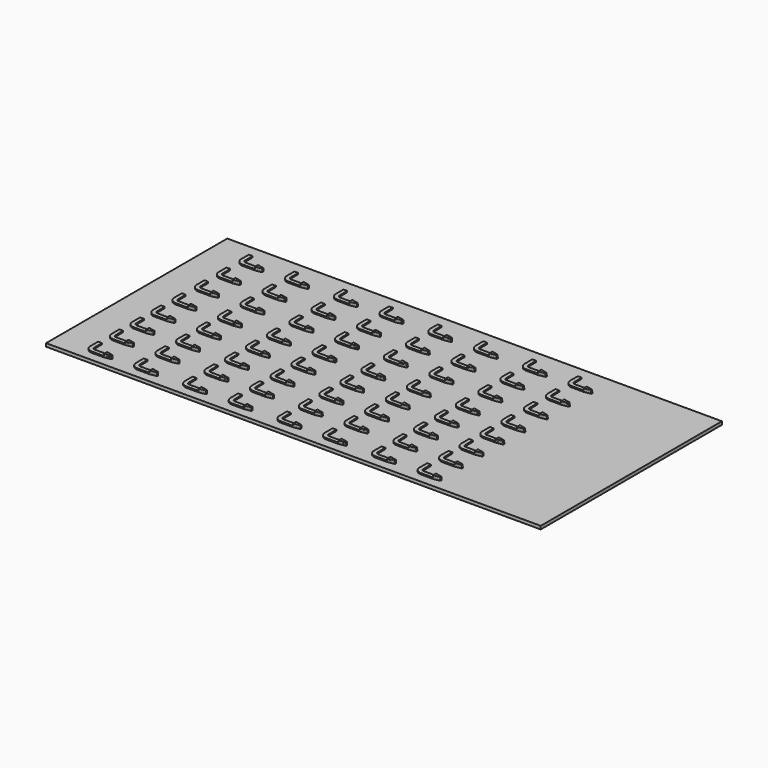
from build123d import *

# Parameters (mm, degrees)
F0_W     = 3907.0630930364
F0_H     = 1789.1258522868
F1_DEPTH = 25.4
F3_DEPTH = 10.16
F5_DEPTH = 7.62
F7_DEPTH = 7.62


# Not quite as in the source:
# - a feature names something its author has since deleted; it is built from what else it names


with BuildPart() as f1:
    # F0 (on Top) → F1 (new body)
    with BuildSketch(Plane.XY):
        with Locations((1503.1844954938, 391.7114809155)):
            Rectangle(F0_W, F0_H)
    extrude(amount=-F1_DEPTH)


with BuildPart() as f3:
    # F2 (on face) → F3 (new body)
    with BuildSketch(Plane.XY):
        with BuildLine():
            Line((0, 4.8675285652), (-51.4132715762, 16.0222817212))
            Line((-51.4132715762, 16.0222817212), (-149.2118090391, 16.0222817212))
            ThreePointArc((-149.2118090391, 16.0222817212), (-163.1179000848, 21.7124932059), (-169.0462678671, 35.5187356472))
            Line((-169.0462678671, 35.5187356472), (-170.3702134564, 112.54149833))
            Line((-170.3702134564, 112.54149833), (-199.8733133078, 112.0343690405))
            Line((-199.8733133078, 112.0343690405), (-199.8733133078, 35.5187356472))
            ThreePointArc((-199.8733133078, 35.5187356472), (-184.8444308949, 0.045176502), (-149.2118090391, -14.602586627))
            Line((-149.2118090391, -14.602586627), (-51.4132715762, -14.602586627))
            Line((-51.4132715762, -14.602586627), (0, -4.8675285652))
            Line((0, -4.8675285652), (0, 4.8675285652))
        make_face()
        with BuildLine():
            Line((0, 210.3862510994), (-51.4132715762, 221.5410042554))
            Line((-51.4132715762, 221.5410042554), (-149.2118090391, 221.5410042554))
            ThreePointArc((-149.2118090391, 221.5410042554), (-163.1179000848, 227.23121574), (-169.0462678671, 241.0374581814))
            Line((-169.0462678671, 241.0374581814), (-170.3702134564, 318.0602208642))
            Line((-170.3702134564, 318.0602208642), (-199.8733133078, 317.5530915746))
            Line((-199.8733133078, 317.5530915746), (-199.8733133078, 241.0374581814))
            ThreePointArc((-199.8733133078, 241.0374581814), (-184.8444308949, 205.5638990362), (-149.2118090391, 190.9161359072))
            Line((-149.2118090391, 190.9161359072), (-51.4132715762, 190.9161359072))
            Line((-51.4132715762, 190.9161359072), (0, 200.651193969))
            Line((0, 200.651193969), (0, 210.3862510994))
        make_face()
        with BuildLine():
            Line((0, -198.6540211365), (-51.4132715762, -187.4992679805))
            Line((-51.4132715762, -187.4992679805), (-149.2118090391, -187.4992679805))
            ThreePointArc((-149.2118090391, -187.4992679805), (-163.1179000848, -181.8090564958), (-169.0462678671, -168.0028140545))
            Line((-169.0462678671, -168.0028140545), (-170.3702134564, -90.9800513717))
            Line((-170.3702134564, -90.9800513717), (-199.8733133078, -91.4871806612))
            Line((-199.8733133078, -91.4871806612), (-199.8733133078, -168.0028140545))
            ThreePointArc((-199.8733133078, -168.0028140545), (-184.8444308949, -203.4763731996), (-149.2118090391, -218.1241363287))
            Line((-149.2118090391, -218.1241363287), (-51.4132715762, -218.1241363287))
            Line((-51.4132715762, -218.1241363287), (0, -208.3890782669))
            Line((0, -208.3890782669), (0, -198.6540211365))
        make_face()
        with BuildLine():
            Line((0, -409.4740850851), (-51.4132715762, -398.3193319291))
            Line((-51.4132715762, -398.3193319291), (-149.2118090391, -398.3193319291))
            ThreePointArc((-149.2118090391, -398.3193319291), (-163.1179000848, -392.6291204445), (-169.0462678671, -378.8228780031))
            Line((-169.0462678671, -378.8228780031), (-170.3702134564, -301.8001153203))
            Line((-170.3702134564, -301.8001153203), (-199.8733133078, -302.3072446099))
            Line((-199.8733133078, -302.3072446099), (-199.8733133078, -378.8228780031))
            ThreePointArc((-199.8733133078, -378.8228780031), (-184.8444308949, -414.2964371483), (-149.2118090391, -428.9442002773))
            Line((-149.2118090391, -428.9442002773), (-51.4132715762, -428.9442002773))
            Line((-51.4132715762, -428.9442002773), (0, -419.2091422155))
            Line((0, -419.2091422155), (0, -409.4740850851))
        make_face()
        with BuildLine():
            Line((0, 418.081481941), (-51.4132715762, 429.2362350971))
            Line((-51.4132715762, 429.2362350971), (-149.2118090391, 429.2362350971))
            ThreePointArc((-149.2118090391, 429.2362350971), (-163.1179000848, 434.9264465817), (-169.0462678671, 448.732689023))
            Line((-169.0462678671, 448.732689023), (-170.3702134564, 525.7554517058))
            Line((-170.3702134564, 525.7554517058), (-199.8733133078, 525.2483224163))
            Line((-199.8733133078, 525.2483224163), (-199.8733133078, 448.732689023))
            ThreePointArc((-199.8733133078, 448.732689023), (-184.8444308949, 413.2591298779), (-149.2118090391, 398.6113667488))
            Line((-149.2118090391, 398.6113667488), (-51.4132715762, 398.6113667488))
            Line((-51.4132715762, 398.6113667488), (0, 408.3464248106))
            Line((0, 408.3464248106), (0, 418.081481941))
        make_face()
        with BuildLine():
            Line((0, 640.5441214507), (-51.4132715762, 651.6988746067))
            Line((-51.4132715762, 651.6988746067), (-149.2118090391, 651.6988746067))
            ThreePointArc((-149.2118090391, 651.6988746067), (-163.1179000848, 657.3890860913), (-169.0462678671, 671.1953285327))
            Line((-169.0462678671, 671.1953285327), (-170.3702134564, 748.2180912155))
            Line((-170.3702134564, 748.2180912155), (-199.8733133078, 747.7109619259))
            Line((-199.8733133078, 747.7109619259), (-199.8733133078, 671.1953285327))
            ThreePointArc((-199.8733133078, 671.1953285327), (-184.8444308949, 635.7217693875), (-149.2118090391, 621.0740062585))
            Line((-149.2118090391, 621.0740062585), (-51.4132715762, 621.0740062585))
            Line((-51.4132715762, 621.0740062585), (0, 630.8090643202))
            Line((0, 630.8090643202), (0, 640.5441214507))
        make_face()
        with BuildLine():
            Line((0, 857.8696446493), (-51.4132715762, 869.0243978053))
            Line((-51.4132715762, 869.0243978053), (-149.2118090391, 869.0243978053))
            ThreePointArc((-149.2118090391, 869.0243978053), (-163.1179000848, 874.71460929), (-169.0462678671, 888.5208517313))
            Line((-169.0462678671, 888.5208517313), (-170.3702134564, 965.5436144141))
            Line((-170.3702134564, 965.5436144141), (-199.8733133078, 965.0364851246))
            Line((-199.8733133078, 965.0364851246), (-199.8733133078, 888.5208517313))
            ThreePointArc((-199.8733133078, 888.5208517313), (-184.8444308949, 853.0472925861), (-149.2118090391, 838.3995294571))
            Line((-149.2118090391, 838.3995294571), (-51.4132715762, 838.3995294571))
            Line((-51.4132715762, 838.3995294571), (0, 848.1345875189))
            Line((0, 848.1345875189), (0, 857.8696446493))
        make_face()
        with BuildLine():
            Line((0, 1078.9936976507), (-51.4132715762, 1090.1484508067))
            Line((-51.4132715762, 1090.1484508067), (-149.2118090391, 1090.1484508067))
            ThreePointArc((-149.2118090391, 1090.1484508067), (-163.1179000848, 1095.8386622914), (-169.0462678671, 1109.6449047327))
            Line((-169.0462678671, 1109.6449047327), (-170.3702134564, 1186.6676674155))
            Line((-170.3702134564, 1186.6676674155), (-199.8733133078, 1186.160538126))
            Line((-199.8733133078, 1186.160538126), (-199.8733133078, 1109.6449047327))
            ThreePointArc((-199.8733133078, 1109.6449047327), (-184.8444308949, 1074.1713455875), (-149.2118090391, 1059.5235824585))
            Line((-149.2118090391, 1059.5235824585), (-51.4132715762, 1059.5235824585))
            Line((-51.4132715762, 1059.5235824585), (0, 1069.2586405203))
            Line((0, 1069.2586405203), (0, 1078.9936976507))
        make_face()
        with BuildLine():
            Line((360.0319474936, 4.8675285652), (308.6186759174, 16.0222817212))
            Line((308.6186759174, 16.0222817212), (210.8201384544, 16.0222817212))
            ThreePointArc((210.8201384544, 16.0222817212), (196.9140474087, 21.7124932059), (190.9856796265, 35.5187356472))
            Line((190.9856796265, 35.5187356472), (189.6617340371, 112.54149833))
            Line((189.6617340371, 112.54149833), (160.1586341858, 112.0343690405))
            Line((160.1586341858, 112.0343690405), (160.1586341858, 35.5187356472))
            ThreePointArc((160.1586341858, 35.5187356472), (175.1875165986, 0.045176502), (210.8201384544, -14.602586627))
            Line((210.8201384544, -14.602586627), (308.6186759174, -14.602586627))
            Line((308.6186759174, -14.602586627), (360.0319474936, -4.8675285652))
            Line((360.0319474936, -4.8675285652), (360.0319474936, 4.8675285652))
        make_face()
        with BuildLine():
            Line((360.0319474936, 210.3862510994), (308.6186759174, 221.5410042554))
            Line((308.6186759174, 221.5410042554), (210.8201384544, 221.5410042554))
            ThreePointArc((210.8201384544, 221.5410042554), (196.9140474087, 227.23121574), (190.9856796265, 241.0374581814))
            Line((190.9856796265, 241.0374581814), (189.6617340371, 318.0602208642))
            Line((189.6617340371, 318.0602208642), (160.1586341858, 317.5530915746))
            Line((160.1586341858, 317.5530915746), (160.1586341858, 241.0374581814))
            ThreePointArc((160.1586341858, 241.0374581814), (175.1875165986, 205.5638990362), (210.8201384544, 190.9161359072))
            Line((210.8201384544, 190.9161359072), (308.6186759174, 190.9161359072))
            Line((308.6186759174, 190.9161359072), (360.0319474936, 200.651193969))
            Line((360.0319474936, 200.651193969), (360.0319474936, 210.3862510994))
        make_face()
        with BuildLine():
            Line((360.0319474936, -198.6540211365), (308.6186759174, -187.4992679805))
            Line((308.6186759174, -187.4992679805), (210.8201384544, -187.4992679805))
            ThreePointArc((210.8201384544, -187.4992679805), (196.9140474087, -181.8090564958), (190.9856796265, -168.0028140545))
            Line((190.9856796265, -168.0028140545), (189.6617340371, -90.9800513717))
            Line((189.6617340371, -90.9800513717), (160.1586341858, -91.4871806612))
            Line((160.1586341858, -91.4871806612), (160.1586341858, -168.0028140545))
            ThreePointArc((160.1586341858, -168.0028140545), (175.1875165986, -203.4763731996), (210.8201384544, -218.1241363287))
            Line((210.8201384544, -218.1241363287), (308.6186759174, -218.1241363287))
            Line((308.6186759174, -218.1241363287), (360.0319474936, -208.3890782669))
            Line((360.0319474936, -208.3890782669), (360.0319474936, -198.6540211365))
        make_face()
        with BuildLine():
            Line((360.0319474936, -409.4740850851), (308.6186759174, -398.3193319291))
            Line((308.6186759174, -398.3193319291), (210.8201384544, -398.3193319291))
            ThreePointArc((210.8201384544, -398.3193319291), (196.9140474087, -392.6291204445), (190.9856796265, -378.8228780031))
            Line((190.9856796265, -378.8228780031), (189.6617340371, -301.8001153203))
            Line((189.6617340371, -301.8001153203), (160.1586341858, -302.3072446099))
            Line((160.1586341858, -302.3072446099), (160.1586341858, -378.8228780031))
            ThreePointArc((160.1586341858, -378.8228780031), (175.1875165986, -414.2964371483), (210.8201384544, -428.9442002773))
            Line((210.8201384544, -428.9442002773), (308.6186759174, -428.9442002773))
            Line((308.6186759174, -428.9442002773), (360.0319474936, -419.2091422155))
            Line((360.0319474936, -419.2091422155), (360.0319474936, -409.4740850851))
        make_face()
        with BuildLine():
            Line((360.0319474936, 418.081481941), (308.6186759174, 429.2362350971))
            Line((308.6186759174, 429.2362350971), (210.8201384544, 429.2362350971))
            ThreePointArc((210.8201384544, 429.2362350971), (196.9140474087, 434.9264465817), (190.9856796265, 448.732689023))
            Line((190.9856796265, 448.732689023), (189.6617340371, 525.7554517058))
            Line((189.6617340371, 525.7554517058), (160.1586341858, 525.2483224163))
            Line((160.1586341858, 525.2483224163), (160.1586341858, 448.732689023))
            ThreePointArc((160.1586341858, 448.732689023), (175.1875165986, 413.2591298779), (210.8201384544, 398.6113667488))
            Line((210.8201384544, 398.6113667488), (308.6186759174, 398.6113667488))
            Line((308.6186759174, 398.6113667488), (360.0319474936, 408.3464248106))
            Line((360.0319474936, 408.3464248106), (360.0319474936, 418.081481941))
        make_face()
        with BuildLine():
            Line((360.0319474936, 640.5441214507), (308.6186759174, 651.6988746067))
            Line((308.6186759174, 651.6988746067), (210.8201384544, 651.6988746067))
            ThreePointArc((210.8201384544, 651.6988746067), (196.9140474087, 657.3890860913), (190.9856796265, 671.1953285327))
            Line((190.9856796265, 671.1953285327), (189.6617340371, 748.2180912155))
            Line((189.6617340371, 748.2180912155), (160.1586341858, 747.7109619259))
            Line((160.1586341858, 747.7109619259), (160.1586341858, 671.1953285327))
            ThreePointArc((160.1586341858, 671.1953285327), (175.1875165986, 635.7217693875), (210.8201384544, 621.0740062585))
            Line((210.8201384544, 621.0740062585), (308.6186759174, 621.0740062585))
            Line((308.6186759174, 621.0740062585), (360.0319474936, 630.8090643202))
            Line((360.0319474936, 630.8090643202), (360.0319474936, 640.5441214507))
        make_face()
        with BuildLine():
            Line((360.0319474936, 857.8696446493), (308.6186759174, 869.0243978053))
            Line((308.6186759174, 869.0243978053), (210.8201384544, 869.0243978053))
            ThreePointArc((210.8201384544, 869.0243978053), (196.9140474087, 874.71460929), (190.9856796265, 888.5208517313))
            Line((190.9856796265, 888.5208517313), (189.6617340371, 965.5436144141))
            Line((189.6617340371, 965.5436144141), (160.1586341858, 965.0364851246))
            Line((160.1586341858, 965.0364851246), (160.1586341858, 888.5208517313))
            ThreePointArc((160.1586341858, 888.5208517313), (175.1875165986, 853.0472925861), (210.8201384544, 838.3995294571))
            Line((210.8201384544, 838.3995294571), (308.6186759174, 838.3995294571))
            Line((308.6186759174, 838.3995294571), (360.0319474936, 848.1345875189))
            Line((360.0319474936, 848.1345875189), (360.0319474936, 857.8696446493))
        make_face()
        with BuildLine():
            Line((360.0319474936, 1078.9936976507), (308.6186759174, 1090.1484508067))
            Line((308.6186759174, 1090.1484508067), (210.8201384544, 1090.1484508067))
            ThreePointArc((210.8201384544, 1090.1484508067), (196.9140474087, 1095.8386622914), (190.9856796265, 1109.6449047327))
            Line((190.9856796265, 1109.6449047327), (189.6617340371, 1186.6676674155))
            Line((189.6617340371, 1186.6676674155), (160.1586341858, 1186.160538126))
            Line((160.1586341858, 1186.160538126), (160.1586341858, 1109.6449047327))
            ThreePointArc((160.1586341858, 1109.6449047327), (175.1875165986, 1074.1713455875), (210.8201384544, 1059.5235824585))
            Line((210.8201384544, 1059.5235824585), (308.6186759174, 1059.5235824585))
            Line((308.6186759174, 1059.5235824585), (360.0319474936, 1069.2586405203))
            Line((360.0319474936, 1069.2586405203), (360.0319474936, 1078.9936976507))
        make_face()
        with BuildLine():
            Line((746.7512339354, 4.8675285652), (695.3379623592, 16.0222817212))
            Line((695.3379623592, 16.0222817212), (597.5394248962, 16.0222817212))
            ThreePointArc((597.5394248962, 16.0222817212), (583.6333338505, 21.7124932059), (577.7049660683, 35.5187356472))
            Line((577.7049660683, 35.5187356472), (576.3810204789, 112.54149833))
            Line((576.3810204789, 112.54149833), (546.8779206276, 112.0343690405))
            Line((546.8779206276, 112.0343690405), (546.8779206276, 35.5187356472))
            ThreePointArc((546.8779206276, 35.5187356472), (561.9068030404, 0.045176502), (597.5394248962, -14.602586627))
            Line((597.5394248962, -14.602586627), (695.3379623592, -14.602586627))
            Line((695.3379623592, -14.602586627), (746.7512339354, -4.8675285652))
            Line((746.7512339354, -4.8675285652), (746.7512339354, 4.8675285652))
        make_face()
        with BuildLine():
            Line((746.7512339354, 210.3862510994), (695.3379623592, 221.5410042554))
            Line((695.3379623592, 221.5410042554), (597.5394248962, 221.5410042554))
            ThreePointArc((597.5394248962, 221.5410042554), (583.6333338505, 227.23121574), (577.7049660683, 241.0374581814))
            Line((577.7049660683, 241.0374581814), (576.3810204789, 318.0602208642))
            Line((576.3810204789, 318.0602208642), (546.8779206276, 317.5530915746))
            Line((546.8779206276, 317.5530915746), (546.8779206276, 241.0374581814))
            ThreePointArc((546.8779206276, 241.0374581814), (561.9068030404, 205.5638990362), (597.5394248962, 190.9161359072))
            Line((597.5394248962, 190.9161359072), (695.3379623592, 190.9161359072))
            Line((695.3379623592, 190.9161359072), (746.7512339354, 200.651193969))
            Line((746.7512339354, 200.651193969), (746.7512339354, 210.3862510994))
        make_face()
        with BuildLine():
            Line((746.7512339354, -198.6540211365), (695.3379623592, -187.4992679805))
            Line((695.3379623592, -187.4992679805), (597.5394248962, -187.4992679805))
            ThreePointArc((597.5394248962, -187.4992679805), (583.6333338505, -181.8090564958), (577.7049660683, -168.0028140545))
            Line((577.7049660683, -168.0028140545), (576.3810204789, -90.9800513717))
            Line((576.3810204789, -90.9800513717), (546.8779206276, -91.4871806612))
            Line((546.8779206276, -91.4871806612), (546.8779206276, -168.0028140545))
            ThreePointArc((546.8779206276, -168.0028140545), (561.9068030404, -203.4763731996), (597.5394248962, -218.1241363287))
            Line((597.5394248962, -218.1241363287), (695.3379623592, -218.1241363287))
            Line((695.3379623592, -218.1241363287), (746.7512339354, -208.3890782669))
            Line((746.7512339354, -208.3890782669), (746.7512339354, -198.6540211365))
        make_face()
        with BuildLine():
            Line((746.7512339354, -409.4740850851), (695.3379623592, -398.3193319291))
            Line((695.3379623592, -398.3193319291), (597.5394248962, -398.3193319291))
            ThreePointArc((597.5394248962, -398.3193319291), (583.6333338505, -392.6291204445), (577.7049660683, -378.8228780031))
            Line((577.7049660683, -378.8228780031), (576.3810204789, -301.8001153203))
            Line((576.3810204789, -301.8001153203), (546.8779206276, -302.3072446099))
            Line((546.8779206276, -302.3072446099), (546.8779206276, -378.8228780031))
            ThreePointArc((546.8779206276, -378.8228780031), (561.9068030404, -414.2964371483), (597.5394248962, -428.9442002773))
            Line((597.5394248962, -428.9442002773), (695.3379623592, -428.9442002773))
            Line((695.3379623592, -428.9442002773), (746.7512339354, -419.2091422155))
            Line((746.7512339354, -419.2091422155), (746.7512339354, -409.4740850851))
        make_face()
        with BuildLine():
            Line((746.7512339354, 418.081481941), (695.3379623592, 429.2362350971))
            Line((695.3379623592, 429.2362350971), (597.5394248962, 429.2362350971))
            ThreePointArc((597.5394248962, 429.2362350971), (583.6333338505, 434.9264465817), (577.7049660683, 448.732689023))
            Line((577.7049660683, 448.732689023), (576.3810204789, 525.7554517058))
            Line((576.3810204789, 525.7554517058), (546.8779206276, 525.2483224163))
            Line((546.8779206276, 525.2483224163), (546.8779206276, 448.732689023))
            ThreePointArc((546.8779206276, 448.732689023), (561.9068030404, 413.2591298779), (597.5394248962, 398.6113667488))
            Line((597.5394248962, 398.6113667488), (695.3379623592, 398.6113667488))
            Line((695.3379623592, 398.6113667488), (746.7512339354, 408.3464248106))
            Line((746.7512339354, 408.3464248106), (746.7512339354, 418.081481941))
        make_face()
        with BuildLine():
            Line((746.7512339354, 640.5441214507), (695.3379623592, 651.6988746067))
            Line((695.3379623592, 651.6988746067), (597.5394248962, 651.6988746067))
            ThreePointArc((597.5394248962, 651.6988746067), (583.6333338505, 657.3890860913), (577.7049660683, 671.1953285327))
            Line((577.7049660683, 671.1953285327), (576.3810204789, 748.2180912155))
            Line((576.3810204789, 748.2180912155), (546.8779206276, 747.7109619259))
            Line((546.8779206276, 747.7109619259), (546.8779206276, 671.1953285327))
            ThreePointArc((546.8779206276, 671.1953285327), (561.9068030404, 635.7217693875), (597.5394248962, 621.0740062585))
            Line((597.5394248962, 621.0740062585), (695.3379623592, 621.0740062585))
            Line((695.3379623592, 621.0740062585), (746.7512339354, 630.8090643202))
            Line((746.7512339354, 630.8090643202), (746.7512339354, 640.5441214507))
        make_face()
        with BuildLine():
            Line((746.7512339354, 857.8696446493), (695.3379623592, 869.0243978053))
            Line((695.3379623592, 869.0243978053), (597.5394248962, 869.0243978053))
            ThreePointArc((597.5394248962, 869.0243978053), (583.6333338505, 874.71460929), (577.7049660683, 888.5208517313))
            Line((577.7049660683, 888.5208517313), (576.3810204789, 965.5436144141))
            Line((576.3810204789, 965.5436144141), (546.8779206276, 965.0364851246))
            Line((546.8779206276, 965.0364851246), (546.8779206276, 888.5208517313))
            ThreePointArc((546.8779206276, 888.5208517313), (561.9068030404, 853.0472925861), (597.5394248962, 838.3995294571))
            Line((597.5394248962, 838.3995294571), (695.3379623592, 838.3995294571))
            Line((695.3379623592, 838.3995294571), (746.7512339354, 848.1345875189))
            Line((746.7512339354, 848.1345875189), (746.7512339354, 857.8696446493))
        make_face()
        with BuildLine():
            Line((746.7512339354, 1078.9936976507), (695.3379623592, 1090.1484508067))
            Line((695.3379623592, 1090.1484508067), (597.5394248962, 1090.1484508067))
            ThreePointArc((597.5394248962, 1090.1484508067), (583.6333338505, 1095.8386622914), (577.7049660683, 1109.6449047327))
            Line((577.7049660683, 1109.6449047327), (576.3810204789, 1186.6676674155))
            Line((576.3810204789, 1186.6676674155), (546.8779206276, 1186.160538126))
            Line((546.8779206276, 1186.160538126), (546.8779206276, 1109.6449047327))
            ThreePointArc((546.8779206276, 1109.6449047327), (561.9068030404, 1074.1713455875), (597.5394248962, 1059.5235824585))
            Line((597.5394248962, 1059.5235824585), (695.3379623592, 1059.5235824585))
            Line((695.3379623592, 1059.5235824585), (746.7512339354, 1069.2586405203))
            Line((746.7512339354, 1069.2586405203), (746.7512339354, 1078.9936976507))
        make_face()
        with BuildLine():
            Line((1106.7831814289, 4.8675285652), (1055.3699098527, 16.0222817212))
            Line((1055.3699098527, 16.0222817212), (957.5713723898, 16.0222817212))
            ThreePointArc((957.5713723898, 16.0222817212), (943.6652813441, 21.7124932059), (937.7369135618, 35.5187356472))
            Line((937.7369135618, 35.5187356472), (936.4129679725, 112.54149833))
            Line((936.4129679725, 112.54149833), (906.9098681211, 112.0343690405))
            Line((906.9098681211, 112.0343690405), (906.9098681211, 35.5187356472))
            ThreePointArc((906.9098681211, 35.5187356472), (921.938750534, 0.045176502), (957.5713723898, -14.602586627))
            Line((957.5713723898, -14.602586627), (1055.3699098527, -14.602586627))
            Line((1055.3699098527, -14.602586627), (1106.7831814289, -4.8675285652))
            Line((1106.7831814289, -4.8675285652), (1106.7831814289, 4.8675285652))
        make_face()
        with BuildLine():
            Line((1106.7831814289, 210.3862510994), (1055.3699098527, 221.5410042554))
            Line((1055.3699098527, 221.5410042554), (957.5713723898, 221.5410042554))
            ThreePointArc((957.5713723898, 221.5410042554), (943.6652813441, 227.23121574), (937.7369135618, 241.0374581814))
            Line((937.7369135618, 241.0374581814), (936.4129679725, 318.0602208642))
            Line((936.4129679725, 318.0602208642), (906.9098681211, 317.5530915746))
            Line((906.9098681211, 317.5530915746), (906.9098681211, 241.0374581814))
            ThreePointArc((906.9098681211, 241.0374581814), (921.938750534, 205.5638990362), (957.5713723898, 190.9161359072))
            Line((957.5713723898, 190.9161359072), (1055.3699098527, 190.9161359072))
            Line((1055.3699098527, 190.9161359072), (1106.7831814289, 200.651193969))
            Line((1106.7831814289, 200.651193969), (1106.7831814289, 210.3862510994))
        make_face()
        with BuildLine():
            Line((1106.7831814289, -198.6540211365), (1055.3699098527, -187.4992679805))
            Line((1055.3699098527, -187.4992679805), (957.5713723898, -187.4992679805))
            ThreePointArc((957.5713723898, -187.4992679805), (943.6652813441, -181.8090564958), (937.7369135618, -168.0028140545))
            Line((937.7369135618, -168.0028140545), (936.4129679725, -90.9800513717))
            Line((936.4129679725, -90.9800513717), (906.9098681211, -91.4871806612))
            Line((906.9098681211, -91.4871806612), (906.9098681211, -168.0028140545))
            ThreePointArc((906.9098681211, -168.0028140545), (921.938750534, -203.4763731996), (957.5713723898, -218.1241363287))
            Line((957.5713723898, -218.1241363287), (1055.3699098527, -218.1241363287))
            Line((1055.3699098527, -218.1241363287), (1106.7831814289, -208.3890782669))
            Line((1106.7831814289, -208.3890782669), (1106.7831814289, -198.6540211365))
        make_face()
        with BuildLine():
            Line((1106.7831814289, -409.4740850851), (1055.3699098527, -398.3193319291))
            Line((1055.3699098527, -398.3193319291), (957.5713723898, -398.3193319291))
            ThreePointArc((957.5713723898, -398.3193319291), (943.6652813441, -392.6291204445), (937.7369135618, -378.8228780031))
            Line((937.7369135618, -378.8228780031), (936.4129679725, -301.8001153203))
            Line((936.4129679725, -301.8001153203), (906.9098681211, -302.3072446099))
            Line((906.9098681211, -302.3072446099), (906.9098681211, -378.8228780031))
            ThreePointArc((906.9098681211, -378.8228780031), (921.938750534, -414.2964371483), (957.5713723898, -428.9442002773))
            Line((957.5713723898, -428.9442002773), (1055.3699098527, -428.9442002773))
            Line((1055.3699098527, -428.9442002773), (1106.7831814289, -419.2091422155))
            Line((1106.7831814289, -419.2091422155), (1106.7831814289, -409.4740850851))
        make_face()
        with BuildLine():
            Line((1106.7831814289, 418.081481941), (1055.3699098527, 429.2362350971))
            Line((1055.3699098527, 429.2362350971), (957.5713723898, 429.2362350971))
            ThreePointArc((957.5713723898, 429.2362350971), (943.6652813441, 434.9264465817), (937.7369135618, 448.732689023))
            Line((937.7369135618, 448.732689023), (936.4129679725, 525.7554517058))
            Line((936.4129679725, 525.7554517058), (906.9098681211, 525.2483224163))
            Line((906.9098681211, 525.2483224163), (906.9098681211, 448.732689023))
            ThreePointArc((906.9098681211, 448.732689023), (921.938750534, 413.2591298779), (957.5713723898, 398.6113667488))
            Line((957.5713723898, 398.6113667488), (1055.3699098527, 398.6113667488))
            Line((1055.3699098527, 398.6113667488), (1106.7831814289, 408.3464248106))
            Line((1106.7831814289, 408.3464248106), (1106.7831814289, 418.081481941))
        make_face()
        with BuildLine():
            Line((1106.7831814289, 640.5441214507), (1055.3699098527, 651.6988746067))
            Line((1055.3699098527, 651.6988746067), (957.5713723898, 651.6988746067))
            ThreePointArc((957.5713723898, 651.6988746067), (943.6652813441, 657.3890860913), (937.7369135618, 671.1953285327))
            Line((937.7369135618, 671.1953285327), (936.4129679725, 748.2180912155))
            Line((936.4129679725, 748.2180912155), (906.9098681211, 747.7109619259))
            Line((906.9098681211, 747.7109619259), (906.9098681211, 671.1953285327))
            ThreePointArc((906.9098681211, 671.1953285327), (921.938750534, 635.7217693875), (957.5713723898, 621.0740062585))
            Line((957.5713723898, 621.0740062585), (1055.3699098527, 621.0740062585))
            Line((1055.3699098527, 621.0740062585), (1106.7831814289, 630.8090643202))
            Line((1106.7831814289, 630.8090643202), (1106.7831814289, 640.5441214507))
        make_face()
        with BuildLine():
            Line((1106.7831814289, 857.8696446493), (1055.3699098527, 869.0243978053))
            Line((1055.3699098527, 869.0243978053), (957.5713723898, 869.0243978053))
            ThreePointArc((957.5713723898, 869.0243978053), (943.6652813441, 874.71460929), (937.7369135618, 888.5208517313))
            Line((937.7369135618, 888.5208517313), (936.4129679725, 965.5436144141))
            Line((936.4129679725, 965.5436144141), (906.9098681211, 965.0364851246))
            Line((906.9098681211, 965.0364851246), (906.9098681211, 888.5208517313))
            ThreePointArc((906.9098681211, 888.5208517313), (921.938750534, 853.0472925861), (957.5713723898, 838.3995294571))
            Line((957.5713723898, 838.3995294571), (1055.3699098527, 838.3995294571))
            Line((1055.3699098527, 838.3995294571), (1106.7831814289, 848.1345875189))
            Line((1106.7831814289, 848.1345875189), (1106.7831814289, 857.8696446493))
        make_face()
        with BuildLine():
            Line((1106.7831814289, 1078.9936976507), (1055.3699098527, 1090.1484508067))
            Line((1055.3699098527, 1090.1484508067), (957.5713723898, 1090.1484508067))
            ThreePointArc((957.5713723898, 1090.1484508067), (943.6652813441, 1095.8386622914), (937.7369135618, 1109.6449047327))
            Line((937.7369135618, 1109.6449047327), (936.4129679725, 1186.6676674155))
            Line((936.4129679725, 1186.6676674155), (906.9098681211, 1186.160538126))
            Line((906.9098681211, 1186.160538126), (906.9098681211, 1109.6449047327))
            ThreePointArc((906.9098681211, 1109.6449047327), (921.938750534, 1074.1713455875), (957.5713723898, 1059.5235824585))
            Line((957.5713723898, 1059.5235824585), (1055.3699098527, 1059.5235824585))
            Line((1055.3699098527, 1059.5235824585), (1106.7831814289, 1069.2586405203))
            Line((1106.7831814289, 1069.2586405203), (1106.7831814289, 1078.9936976507))
        make_face()
        with BuildLine():
            Line((1492.2146052122, 4.8675285652), (1440.801333636, 16.0222817212))
            Line((1440.801333636, 16.0222817212), (1343.0027961731, 16.0222817212))
            ThreePointArc((1343.0027961731, 16.0222817212), (1329.0967051274, 21.7124932059), (1323.1683373451, 35.5187356472))
            Line((1323.1683373451, 35.5187356472), (1321.8443917558, 112.54149833))
            Line((1321.8443917558, 112.54149833), (1292.3412919044, 112.0343690405))
            Line((1292.3412919044, 112.0343690405), (1292.3412919044, 35.5187356472))
            ThreePointArc((1292.3412919044, 35.5187356472), (1307.3701743173, 0.045176502), (1343.0027961731, -14.602586627))
            Line((1343.0027961731, -14.602586627), (1440.801333636, -14.602586627))
            Line((1440.801333636, -14.602586627), (1492.2146052122, -4.8675285652))
            Line((1492.2146052122, -4.8675285652), (1492.2146052122, 4.8675285652))
        make_face()
        with BuildLine():
            Line((1492.2146052122, 210.3862510994), (1440.801333636, 221.5410042554))
            Line((1440.801333636, 221.5410042554), (1343.0027961731, 221.5410042554))
            ThreePointArc((1343.0027961731, 221.5410042554), (1329.0967051274, 227.23121574), (1323.1683373451, 241.0374581814))
            Line((1323.1683373451, 241.0374581814), (1321.8443917558, 318.0602208642))
            Line((1321.8443917558, 318.0602208642), (1292.3412919044, 317.5530915746))
            Line((1292.3412919044, 317.5530915746), (1292.3412919044, 241.0374581814))
            ThreePointArc((1292.3412919044, 241.0374581814), (1307.3701743173, 205.5638990362), (1343.0027961731, 190.9161359072))
            Line((1343.0027961731, 190.9161359072), (1440.801333636, 190.9161359072))
            Line((1440.801333636, 190.9161359072), (1492.2146052122, 200.651193969))
            Line((1492.2146052122, 200.651193969), (1492.2146052122, 210.3862510994))
        make_face()
        with BuildLine():
            Line((1492.2146052122, -198.6540211365), (1440.801333636, -187.4992679805))
            Line((1440.801333636, -187.4992679805), (1343.0027961731, -187.4992679805))
            ThreePointArc((1343.0027961731, -187.4992679805), (1329.0967051274, -181.8090564958), (1323.1683373451, -168.0028140545))
            Line((1323.1683373451, -168.0028140545), (1321.8443917558, -90.9800513717))
            Line((1321.8443917558, -90.9800513717), (1292.3412919044, -91.4871806612))
            Line((1292.3412919044, -91.4871806612), (1292.3412919044, -168.0028140545))
            ThreePointArc((1292.3412919044, -168.0028140545), (1307.3701743173, -203.4763731996), (1343.0027961731, -218.1241363287))
            Line((1343.0027961731, -218.1241363287), (1440.801333636, -218.1241363287))
            Line((1440.801333636, -218.1241363287), (1492.2146052122, -208.3890782669))
            Line((1492.2146052122, -208.3890782669), (1492.2146052122, -198.6540211365))
        make_face()
        with BuildLine():
            Line((1492.2146052122, -409.4740850851), (1440.801333636, -398.3193319291))
            Line((1440.801333636, -398.3193319291), (1343.0027961731, -398.3193319291))
            ThreePointArc((1343.0027961731, -398.3193319291), (1329.0967051274, -392.6291204445), (1323.1683373451, -378.8228780031))
            Line((1323.1683373451, -378.8228780031), (1321.8443917558, -301.8001153203))
            Line((1321.8443917558, -301.8001153203), (1292.3412919044, -302.3072446099))
            Line((1292.3412919044, -302.3072446099), (1292.3412919044, -378.8228780031))
            ThreePointArc((1292.3412919044, -378.8228780031), (1307.3701743173, -414.2964371483), (1343.0027961731, -428.9442002773))
            Line((1343.0027961731, -428.9442002773), (1440.801333636, -428.9442002773))
            Line((1440.801333636, -428.9442002773), (1492.2146052122, -419.2091422155))
            Line((1492.2146052122, -419.2091422155), (1492.2146052122, -409.4740850851))
        make_face()
        with BuildLine():
            Line((1492.2146052122, 418.081481941), (1440.801333636, 429.2362350971))
            Line((1440.801333636, 429.2362350971), (1343.0027961731, 429.2362350971))
            ThreePointArc((1343.0027961731, 429.2362350971), (1329.0967051274, 434.9264465817), (1323.1683373451, 448.732689023))
            Line((1323.1683373451, 448.732689023), (1321.8443917558, 525.7554517058))
            Line((1321.8443917558, 525.7554517058), (1292.3412919044, 525.2483224163))
            Line((1292.3412919044, 525.2483224163), (1292.3412919044, 448.732689023))
            ThreePointArc((1292.3412919044, 448.732689023), (1307.3701743173, 413.2591298779), (1343.0027961731, 398.6113667488))
            Line((1343.0027961731, 398.6113667488), (1440.801333636, 398.6113667488))
            Line((1440.801333636, 398.6113667488), (1492.2146052122, 408.3464248106))
            Line((1492.2146052122, 408.3464248106), (1492.2146052122, 418.081481941))
        make_face()
        with BuildLine():
            Line((1492.2146052122, 640.5441214507), (1440.801333636, 651.6988746067))
            Line((1440.801333636, 651.6988746067), (1343.0027961731, 651.6988746067))
            ThreePointArc((1343.0027961731, 651.6988746067), (1329.0967051274, 657.3890860913), (1323.1683373451, 671.1953285327))
            Line((1323.1683373451, 671.1953285327), (1321.8443917558, 748.2180912155))
            Line((1321.8443917558, 748.2180912155), (1292.3412919044, 747.7109619259))
            Line((1292.3412919044, 747.7109619259), (1292.3412919044, 671.1953285327))
            ThreePointArc((1292.3412919044, 671.1953285327), (1307.3701743173, 635.7217693875), (1343.0027961731, 621.0740062585))
            Line((1343.0027961731, 621.0740062585), (1440.801333636, 621.0740062585))
            Line((1440.801333636, 621.0740062585), (1492.2146052122, 630.8090643202))
            Line((1492.2146052122, 630.8090643202), (1492.2146052122, 640.5441214507))
        make_face()
        with BuildLine():
            Line((1492.2146052122, 857.8696446493), (1440.801333636, 869.0243978053))
            Line((1440.801333636, 869.0243978053), (1343.0027961731, 869.0243978053))
            ThreePointArc((1343.0027961731, 869.0243978053), (1329.0967051274, 874.71460929), (1323.1683373451, 888.5208517313))
            Line((1323.1683373451, 888.5208517313), (1321.8443917558, 965.5436144141))
            Line((1321.8443917558, 965.5436144141), (1292.3412919044, 965.0364851246))
            Line((1292.3412919044, 965.0364851246), (1292.3412919044, 888.5208517313))
            ThreePointArc((1292.3412919044, 888.5208517313), (1307.3701743173, 853.0472925861), (1343.0027961731, 838.3995294571))
            Line((1343.0027961731, 838.3995294571), (1440.801333636, 838.3995294571))
            Line((1440.801333636, 838.3995294571), (1492.2146052122, 848.1345875189))
            Line((1492.2146052122, 848.1345875189), (1492.2146052122, 857.8696446493))
        make_face()
        with BuildLine():
            Line((1492.2146052122, 1078.9936976507), (1440.801333636, 1090.1484508067))
            Line((1440.801333636, 1090.1484508067), (1343.0027961731, 1090.1484508067))
            ThreePointArc((1343.0027961731, 1090.1484508067), (1329.0967051274, 1095.8386622914), (1323.1683373451, 1109.6449047327))
            Line((1323.1683373451, 1109.6449047327), (1321.8443917558, 1186.6676674155))
            Line((1321.8443917558, 1186.6676674155), (1292.3412919044, 1186.160538126))
            Line((1292.3412919044, 1186.160538126), (1292.3412919044, 1109.6449047327))
            ThreePointArc((1292.3412919044, 1109.6449047327), (1307.3701743173, 1074.1713455875), (1343.0027961731, 1059.5235824585))
            Line((1343.0027961731, 1059.5235824585), (1440.801333636, 1059.5235824585))
            Line((1440.801333636, 1059.5235824585), (1492.2146052122, 1069.2586405203))
            Line((1492.2146052122, 1069.2586405203), (1492.2146052122, 1078.9936976507))
        make_face()
        with BuildLine():
            Line((1852.2465527058, 4.8675285652), (1800.8332811296, 16.0222817212))
            Line((1800.8332811296, 16.0222817212), (1703.0347436666, 16.0222817212))
            ThreePointArc((1703.0347436666, 16.0222817212), (1689.1286526209, 21.7124932059), (1683.2002848387, 35.5187356472))
            Line((1683.2002848387, 35.5187356472), (1681.8763392493, 112.54149833))
            Line((1681.8763392493, 112.54149833), (1652.373239398, 112.0343690405))
            Line((1652.373239398, 112.0343690405), (1652.373239398, 35.5187356472))
            ThreePointArc((1652.373239398, 35.5187356472), (1667.4021218108, 0.045176502), (1703.0347436666, -14.602586627))
            Line((1703.0347436666, -14.602586627), (1800.8332811296, -14.602586627))
            Line((1800.8332811296, -14.602586627), (1852.2465527058, -4.8675285652))
            Line((1852.2465527058, -4.8675285652), (1852.2465527058, 4.8675285652))
        make_face()
        with BuildLine():
            Line((1852.2465527058, 210.3862510994), (1800.8332811296, 221.5410042554))
            Line((1800.8332811296, 221.5410042554), (1703.0347436666, 221.5410042554))
            ThreePointArc((1703.0347436666, 221.5410042554), (1689.1286526209, 227.23121574), (1683.2002848387, 241.0374581814))
            Line((1683.2002848387, 241.0374581814), (1681.8763392493, 318.0602208642))
            Line((1681.8763392493, 318.0602208642), (1652.373239398, 317.5530915746))
            Line((1652.373239398, 317.5530915746), (1652.373239398, 241.0374581814))
            ThreePointArc((1652.373239398, 241.0374581814), (1667.4021218108, 205.5638990362), (1703.0347436666, 190.9161359072))
            Line((1703.0347436666, 190.9161359072), (1800.8332811296, 190.9161359072))
            Line((1800.8332811296, 190.9161359072), (1852.2465527058, 200.651193969))
            Line((1852.2465527058, 200.651193969), (1852.2465527058, 210.3862510994))
        make_face()
        with BuildLine():
            Line((1852.2465527058, -198.6540211365), (1800.8332811296, -187.4992679805))
            Line((1800.8332811296, -187.4992679805), (1703.0347436666, -187.4992679805))
            ThreePointArc((1703.0347436666, -187.4992679805), (1689.1286526209, -181.8090564958), (1683.2002848387, -168.0028140545))
            Line((1683.2002848387, -168.0028140545), (1681.8763392493, -90.9800513717))
            Line((1681.8763392493, -90.9800513717), (1652.373239398, -91.4871806612))
            Line((1652.373239398, -91.4871806612), (1652.373239398, -168.0028140545))
            ThreePointArc((1652.373239398, -168.0028140545), (1667.4021218108, -203.4763731996), (1703.0347436666, -218.1241363287))
            Line((1703.0347436666, -218.1241363287), (1800.8332811296, -218.1241363287))
            Line((1800.8332811296, -218.1241363287), (1852.2465527058, -208.3890782669))
            Line((1852.2465527058, -208.3890782669), (1852.2465527058, -198.6540211365))
        make_face()
        with BuildLine():
            Line((1852.2465527058, -409.4740850851), (1800.8332811296, -398.3193319291))
            Line((1800.8332811296, -398.3193319291), (1703.0347436666, -398.3193319291))
            ThreePointArc((1703.0347436666, -398.3193319291), (1689.1286526209, -392.6291204445), (1683.2002848387, -378.8228780031))
            Line((1683.2002848387, -378.8228780031), (1681.8763392493, -301.8001153203))
            Line((1681.8763392493, -301.8001153203), (1652.373239398, -302.3072446099))
            Line((1652.373239398, -302.3072446099), (1652.373239398, -378.8228780031))
            ThreePointArc((1652.373239398, -378.8228780031), (1667.4021218108, -414.2964371483), (1703.0347436666, -428.9442002773))
            Line((1703.0347436666, -428.9442002773), (1800.8332811296, -428.9442002773))
            Line((1800.8332811296, -428.9442002773), (1852.2465527058, -419.2091422155))
            Line((1852.2465527058, -419.2091422155), (1852.2465527058, -409.4740850851))
        make_face()
        with BuildLine():
            Line((1852.2465527058, 418.081481941), (1800.8332811296, 429.2362350971))
            Line((1800.8332811296, 429.2362350971), (1703.0347436666, 429.2362350971))
            ThreePointArc((1703.0347436666, 429.2362350971), (1689.1286526209, 434.9264465817), (1683.2002848387, 448.732689023))
            Line((1683.2002848387, 448.732689023), (1681.8763392493, 525.7554517058))
            Line((1681.8763392493, 525.7554517058), (1652.373239398, 525.2483224163))
            Line((1652.373239398, 525.2483224163), (1652.373239398, 448.732689023))
            ThreePointArc((1652.373239398, 448.732689023), (1667.4021218108, 413.2591298779), (1703.0347436666, 398.6113667488))
            Line((1703.0347436666, 398.6113667488), (1800.8332811296, 398.6113667488))
            Line((1800.8332811296, 398.6113667488), (1852.2465527058, 408.3464248106))
            Line((1852.2465527058, 408.3464248106), (1852.2465527058, 418.081481941))
        make_face()
        with BuildLine():
            Line((1852.2465527058, 640.5441214507), (1800.8332811296, 651.6988746067))
            Line((1800.8332811296, 651.6988746067), (1703.0347436666, 651.6988746067))
            ThreePointArc((1703.0347436666, 651.6988746067), (1689.1286526209, 657.3890860913), (1683.2002848387, 671.1953285327))
            Line((1683.2002848387, 671.1953285327), (1681.8763392493, 748.2180912155))
            Line((1681.8763392493, 748.2180912155), (1652.373239398, 747.7109619259))
            Line((1652.373239398, 747.7109619259), (1652.373239398, 671.1953285327))
            ThreePointArc((1652.373239398, 671.1953285327), (1667.4021218108, 635.7217693875), (1703.0347436666, 621.0740062585))
            Line((1703.0347436666, 621.0740062585), (1800.8332811296, 621.0740062585))
            Line((1800.8332811296, 621.0740062585), (1852.2465527058, 630.8090643202))
            Line((1852.2465527058, 630.8090643202), (1852.2465527058, 640.5441214507))
        make_face()
        with BuildLine():
            Line((1852.2465527058, 857.8696446493), (1800.8332811296, 869.0243978053))
            Line((1800.8332811296, 869.0243978053), (1703.0347436666, 869.0243978053))
            ThreePointArc((1703.0347436666, 869.0243978053), (1689.1286526209, 874.71460929), (1683.2002848387, 888.5208517313))
            Line((1683.2002848387, 888.5208517313), (1681.8763392493, 965.5436144141))
            Line((1681.8763392493, 965.5436144141), (1652.373239398, 965.0364851246))
            Line((1652.373239398, 965.0364851246), (1652.373239398, 888.5208517313))
            ThreePointArc((1652.373239398, 888.5208517313), (1667.4021218108, 853.0472925861), (1703.0347436666, 838.3995294571))
            Line((1703.0347436666, 838.3995294571), (1800.8332811296, 838.3995294571))
            Line((1800.8332811296, 838.3995294571), (1852.2465527058, 848.1345875189))
            Line((1852.2465527058, 848.1345875189), (1852.2465527058, 857.8696446493))
        make_face()
        with BuildLine():
            Line((1852.2465527058, 1078.9936976507), (1800.8332811296, 1090.1484508067))
            Line((1800.8332811296, 1090.1484508067), (1703.0347436666, 1090.1484508067))
            ThreePointArc((1703.0347436666, 1090.1484508067), (1689.1286526209, 1095.8386622914), (1683.2002848387, 1109.6449047327))
            Line((1683.2002848387, 1109.6449047327), (1681.8763392493, 1186.6676674155))
            Line((1681.8763392493, 1186.6676674155), (1652.373239398, 1186.160538126))
            Line((1652.373239398, 1186.160538126), (1652.373239398, 1109.6449047327))
            ThreePointArc((1652.373239398, 1109.6449047327), (1667.4021218108, 1074.1713455875), (1703.0347436666, 1059.5235824585))
            Line((1703.0347436666, 1059.5235824585), (1800.8332811296, 1059.5235824585))
            Line((1800.8332811296, 1059.5235824585), (1852.2465527058, 1069.2586405203))
            Line((1852.2465527058, 1069.2586405203), (1852.2465527058, 1078.9936976507))
        make_face()
        with BuildLine():
            Line((2238.9658391476, 4.8675285652), (2187.5525675714, 16.0222817212))
            Line((2187.5525675714, 16.0222817212), (2089.7540301085, 16.0222817212))
            ThreePointArc((2089.7540301085, 16.0222817212), (2075.8479390627, 21.7124932059), (2069.9195712805, 35.5187356472))
            Line((2069.9195712805, 35.5187356472), (2068.5956256911, 112.54149833))
            Line((2068.5956256911, 112.54149833), (2039.0925258398, 112.0343690405))
            Line((2039.0925258398, 112.0343690405), (2039.0925258398, 35.5187356472))
            ThreePointArc((2039.0925258398, 35.5187356472), (2054.1214082526, 0.045176502), (2089.7540301085, -14.602586627))
            Line((2089.7540301085, -14.602586627), (2187.5525675714, -14.602586627))
            Line((2187.5525675714, -14.602586627), (2238.9658391476, -4.8675285652))
            Line((2238.9658391476, -4.8675285652), (2238.9658391476, 4.8675285652))
        make_face()
        with BuildLine():
            Line((2238.9658391476, 210.3862510994), (2187.5525675714, 221.5410042554))
            Line((2187.5525675714, 221.5410042554), (2089.7540301085, 221.5410042554))
            ThreePointArc((2089.7540301085, 221.5410042554), (2075.8479390627, 227.23121574), (2069.9195712805, 241.0374581814))
            Line((2069.9195712805, 241.0374581814), (2068.5956256911, 318.0602208642))
            Line((2068.5956256911, 318.0602208642), (2039.0925258398, 317.5530915746))
            Line((2039.0925258398, 317.5530915746), (2039.0925258398, 241.0374581814))
            ThreePointArc((2039.0925258398, 241.0374581814), (2054.1214082526, 205.5638990362), (2089.7540301085, 190.9161359072))
            Line((2089.7540301085, 190.9161359072), (2187.5525675714, 190.9161359072))
            Line((2187.5525675714, 190.9161359072), (2238.9658391476, 200.651193969))
            Line((2238.9658391476, 200.651193969), (2238.9658391476, 210.3862510994))
        make_face()
        with BuildLine():
            Line((2238.9658391476, -198.6540211365), (2187.5525675714, -187.4992679805))
            Line((2187.5525675714, -187.4992679805), (2089.7540301085, -187.4992679805))
            ThreePointArc((2089.7540301085, -187.4992679805), (2075.8479390627, -181.8090564958), (2069.9195712805, -168.0028140545))
            Line((2069.9195712805, -168.0028140545), (2068.5956256911, -90.9800513717))
            Line((2068.5956256911, -90.9800513717), (2039.0925258398, -91.4871806612))
            Line((2039.0925258398, -91.4871806612), (2039.0925258398, -168.0028140545))
            ThreePointArc((2039.0925258398, -168.0028140545), (2054.1214082526, -203.4763731996), (2089.7540301085, -218.1241363287))
            Line((2089.7540301085, -218.1241363287), (2187.5525675714, -218.1241363287))
            Line((2187.5525675714, -218.1241363287), (2238.9658391476, -208.3890782669))
            Line((2238.9658391476, -208.3890782669), (2238.9658391476, -198.6540211365))
        make_face()
        with BuildLine():
            Line((2238.9658391476, -409.4740850851), (2187.5525675714, -398.3193319291))
            Line((2187.5525675714, -398.3193319291), (2089.7540301085, -398.3193319291))
            ThreePointArc((2089.7540301085, -398.3193319291), (2075.8479390627, -392.6291204445), (2069.9195712805, -378.8228780031))
            Line((2069.9195712805, -378.8228780031), (2068.5956256911, -301.8001153203))
            Line((2068.5956256911, -301.8001153203), (2039.0925258398, -302.3072446099))
            Line((2039.0925258398, -302.3072446099), (2039.0925258398, -378.8228780031))
            ThreePointArc((2039.0925258398, -378.8228780031), (2054.1214082526, -414.2964371483), (2089.7540301085, -428.9442002773))
            Line((2089.7540301085, -428.9442002773), (2187.5525675714, -428.9442002773))
            Line((2187.5525675714, -428.9442002773), (2238.9658391476, -419.2091422155))
            Line((2238.9658391476, -419.2091422155), (2238.9658391476, -409.4740850851))
        make_face()
        with BuildLine():
            Line((2238.9658391476, 418.081481941), (2187.5525675714, 429.2362350971))
            Line((2187.5525675714, 429.2362350971), (2089.7540301085, 429.2362350971))
            ThreePointArc((2089.7540301085, 429.2362350971), (2075.8479390627, 434.9264465817), (2069.9195712805, 448.732689023))
            Line((2069.9195712805, 448.732689023), (2068.5956256911, 525.7554517058))
            Line((2068.5956256911, 525.7554517058), (2039.0925258398, 525.2483224163))
            Line((2039.0925258398, 525.2483224163), (2039.0925258398, 448.732689023))
            ThreePointArc((2039.0925258398, 448.732689023), (2054.1214082526, 413.2591298779), (2089.7540301085, 398.6113667488))
            Line((2089.7540301085, 398.6113667488), (2187.5525675714, 398.6113667488))
            Line((2187.5525675714, 398.6113667488), (2238.9658391476, 408.3464248106))
            Line((2238.9658391476, 408.3464248106), (2238.9658391476, 418.081481941))
        make_face()
        with BuildLine():
            Line((2238.9658391476, 640.5441214507), (2187.5525675714, 651.6988746067))
            Line((2187.5525675714, 651.6988746067), (2089.7540301085, 651.6988746067))
            ThreePointArc((2089.7540301085, 651.6988746067), (2075.8479390627, 657.3890860913), (2069.9195712805, 671.1953285327))
            Line((2069.9195712805, 671.1953285327), (2068.5956256911, 748.2180912155))
            Line((2068.5956256911, 748.2180912155), (2039.0925258398, 747.7109619259))
            Line((2039.0925258398, 747.7109619259), (2039.0925258398, 671.1953285327))
            ThreePointArc((2039.0925258398, 671.1953285327), (2054.1214082526, 635.7217693875), (2089.7540301085, 621.0740062585))
            Line((2089.7540301085, 621.0740062585), (2187.5525675714, 621.0740062585))
            Line((2187.5525675714, 621.0740062585), (2238.9658391476, 630.8090643202))
            Line((2238.9658391476, 630.8090643202), (2238.9658391476, 640.5441214507))
        make_face()
        with BuildLine():
            Line((2238.9658391476, 857.8696446493), (2187.5525675714, 869.0243978053))
            Line((2187.5525675714, 869.0243978053), (2089.7540301085, 869.0243978053))
            ThreePointArc((2089.7540301085, 869.0243978053), (2075.8479390627, 874.71460929), (2069.9195712805, 888.5208517313))
            Line((2069.9195712805, 888.5208517313), (2068.5956256911, 965.5436144141))
            Line((2068.5956256911, 965.5436144141), (2039.0925258398, 965.0364851246))
            Line((2039.0925258398, 965.0364851246), (2039.0925258398, 888.5208517313))
            ThreePointArc((2039.0925258398, 888.5208517313), (2054.1214082526, 853.0472925861), (2089.7540301085, 838.3995294571))
            Line((2089.7540301085, 838.3995294571), (2187.5525675714, 838.3995294571))
            Line((2187.5525675714, 838.3995294571), (2238.9658391476, 848.1345875189))
            Line((2238.9658391476, 848.1345875189), (2238.9658391476, 857.8696446493))
        make_face()
        with BuildLine():
            Line((2238.9658391476, 1078.9936976507), (2187.5525675714, 1090.1484508067))
            Line((2187.5525675714, 1090.1484508067), (2089.7540301085, 1090.1484508067))
            ThreePointArc((2089.7540301085, 1090.1484508067), (2075.8479390627, 1095.8386622914), (2069.9195712805, 1109.6449047327))
            Line((2069.9195712805, 1109.6449047327), (2068.5956256911, 1186.6676674155))
            Line((2068.5956256911, 1186.6676674155), (2039.0925258398, 1186.160538126))
            Line((2039.0925258398, 1186.160538126), (2039.0925258398, 1109.6449047327))
            ThreePointArc((2039.0925258398, 1109.6449047327), (2054.1214082526, 1074.1713455875), (2089.7540301085, 1059.5235824585))
            Line((2089.7540301085, 1059.5235824585), (2187.5525675714, 1059.5235824585))
            Line((2187.5525675714, 1059.5235824585), (2238.9658391476, 1069.2586405203))
            Line((2238.9658391476, 1069.2586405203), (2238.9658391476, 1078.9936976507))
        make_face()
        with BuildLine():
            Line((2598.9977866411, 4.8675285652), (2547.584515065, 16.0222817212))
            Line((2547.584515065, 16.0222817212), (2449.785977602, 16.0222817212))
            ThreePointArc((2449.785977602, 16.0222817212), (2435.8798865563, 21.7124932059), (2429.951518774, 35.5187356472))
            Line((2429.951518774, 35.5187356472), (2428.6275731847, 112.54149833))
            Line((2428.6275731847, 112.54149833), (2399.1244733334, 112.0343690405))
            Line((2399.1244733334, 112.0343690405), (2399.1244733334, 35.5187356472))
            ThreePointArc((2399.1244733334, 35.5187356472), (2414.1533557462, 0.045176502), (2449.785977602, -14.602586627))
            Line((2449.785977602, -14.602586627), (2547.584515065, -14.602586627))
            Line((2547.584515065, -14.602586627), (2598.9977866411, -4.8675285652))
            Line((2598.9977866411, -4.8675285652), (2598.9977866411, 4.8675285652))
        make_face()
        with BuildLine():
            Line((2598.9977866411, 210.3862510994), (2547.584515065, 221.5410042554))
            Line((2547.584515065, 221.5410042554), (2449.785977602, 221.5410042554))
            ThreePointArc((2449.785977602, 221.5410042554), (2435.8798865563, 227.23121574), (2429.951518774, 241.0374581814))
            Line((2429.951518774, 241.0374581814), (2428.6275731847, 318.0602208642))
            Line((2428.6275731847, 318.0602208642), (2399.1244733334, 317.5530915746))
            Line((2399.1244733334, 317.5530915746), (2399.1244733334, 241.0374581814))
            ThreePointArc((2399.1244733334, 241.0374581814), (2414.1533557462, 205.5638990362), (2449.785977602, 190.9161359072))
            Line((2449.785977602, 190.9161359072), (2547.584515065, 190.9161359072))
            Line((2547.584515065, 190.9161359072), (2598.9977866411, 200.651193969))
            Line((2598.9977866411, 200.651193969), (2598.9977866411, 210.3862510994))
        make_face()
        with BuildLine():
            Line((2598.9977866411, -198.6540211365), (2547.584515065, -187.4992679805))
            Line((2547.584515065, -187.4992679805), (2449.785977602, -187.4992679805))
            ThreePointArc((2449.785977602, -187.4992679805), (2435.8798865563, -181.8090564958), (2429.951518774, -168.0028140545))
            Line((2429.951518774, -168.0028140545), (2428.6275731847, -90.9800513717))
            Line((2428.6275731847, -90.9800513717), (2399.1244733334, -91.4871806612))
            Line((2399.1244733334, -91.4871806612), (2399.1244733334, -168.0028140545))
            ThreePointArc((2399.1244733334, -168.0028140545), (2414.1533557462, -203.4763731996), (2449.785977602, -218.1241363287))
            Line((2449.785977602, -218.1241363287), (2547.584515065, -218.1241363287))
            Line((2547.584515065, -218.1241363287), (2598.9977866411, -208.3890782669))
            Line((2598.9977866411, -208.3890782669), (2598.9977866411, -198.6540211365))
        make_face()
        with BuildLine():
            Line((2598.9977866411, -409.4740850851), (2547.584515065, -398.3193319291))
            Line((2547.584515065, -398.3193319291), (2449.785977602, -398.3193319291))
            ThreePointArc((2449.785977602, -398.3193319291), (2435.8798865563, -392.6291204445), (2429.951518774, -378.8228780031))
            Line((2429.951518774, -378.8228780031), (2428.6275731847, -301.8001153203))
            Line((2428.6275731847, -301.8001153203), (2399.1244733334, -302.3072446099))
            Line((2399.1244733334, -302.3072446099), (2399.1244733334, -378.8228780031))
            ThreePointArc((2399.1244733334, -378.8228780031), (2414.1533557462, -414.2964371483), (2449.785977602, -428.9442002773))
            Line((2449.785977602, -428.9442002773), (2547.584515065, -428.9442002773))
            Line((2547.584515065, -428.9442002773), (2598.9977866411, -419.2091422155))
            Line((2598.9977866411, -419.2091422155), (2598.9977866411, -409.4740850851))
        make_face()
        with BuildLine():
            Line((2598.9977866411, 418.081481941), (2547.584515065, 429.2362350971))
            Line((2547.584515065, 429.2362350971), (2449.785977602, 429.2362350971))
            ThreePointArc((2449.785977602, 429.2362350971), (2435.8798865563, 434.9264465817), (2429.951518774, 448.732689023))
            Line((2429.951518774, 448.732689023), (2428.6275731847, 525.7554517058))
            Line((2428.6275731847, 525.7554517058), (2399.1244733334, 525.2483224163))
            Line((2399.1244733334, 525.2483224163), (2399.1244733334, 448.732689023))
            ThreePointArc((2399.1244733334, 448.732689023), (2414.1533557462, 413.2591298779), (2449.785977602, 398.6113667488))
            Line((2449.785977602, 398.6113667488), (2547.584515065, 398.6113667488))
            Line((2547.584515065, 398.6113667488), (2598.9977866411, 408.3464248106))
            Line((2598.9977866411, 408.3464248106), (2598.9977866411, 418.081481941))
        make_face()
        with BuildLine():
            Line((2598.9977866411, 640.5441214507), (2547.584515065, 651.6988746067))
            Line((2547.584515065, 651.6988746067), (2449.785977602, 651.6988746067))
            ThreePointArc((2449.785977602, 651.6988746067), (2435.8798865563, 657.3890860913), (2429.951518774, 671.1953285327))
            Line((2429.951518774, 671.1953285327), (2428.6275731847, 748.2180912155))
            Line((2428.6275731847, 748.2180912155), (2399.1244733334, 747.7109619259))
            Line((2399.1244733334, 747.7109619259), (2399.1244733334, 671.1953285327))
            ThreePointArc((2399.1244733334, 671.1953285327), (2414.1533557462, 635.7217693875), (2449.785977602, 621.0740062585))
            Line((2449.785977602, 621.0740062585), (2547.584515065, 621.0740062585))
            Line((2547.584515065, 621.0740062585), (2598.9977866411, 630.8090643202))
            Line((2598.9977866411, 630.8090643202), (2598.9977866411, 640.5441214507))
        make_face()
        with BuildLine():
            Line((2598.9977866411, 857.8696446493), (2547.584515065, 869.0243978053))
            Line((2547.584515065, 869.0243978053), (2449.785977602, 869.0243978053))
            ThreePointArc((2449.785977602, 869.0243978053), (2435.8798865563, 874.71460929), (2429.951518774, 888.5208517313))
            Line((2429.951518774, 888.5208517313), (2428.6275731847, 965.5436144141))
            Line((2428.6275731847, 965.5436144141), (2399.1244733334, 965.0364851246))
            Line((2399.1244733334, 965.0364851246), (2399.1244733334, 888.5208517313))
            ThreePointArc((2399.1244733334, 888.5208517313), (2414.1533557462, 853.0472925861), (2449.785977602, 838.3995294571))
            Line((2449.785977602, 838.3995294571), (2547.584515065, 838.3995294571))
            Line((2547.584515065, 838.3995294571), (2598.9977866411, 848.1345875189))
            Line((2598.9977866411, 848.1345875189), (2598.9977866411, 857.8696446493))
        make_face()
        with BuildLine():
            Line((2598.9977866411, 1078.9936976507), (2547.584515065, 1090.1484508067))
            Line((2547.584515065, 1090.1484508067), (2449.785977602, 1090.1484508067))
            ThreePointArc((2449.785977602, 1090.1484508067), (2435.8798865563, 1095.8386622914), (2429.951518774, 1109.6449047327))
            Line((2429.951518774, 1109.6449047327), (2428.6275731847, 1186.6676674155))
            Line((2428.6275731847, 1186.6676674155), (2399.1244733334, 1186.160538126))
            Line((2399.1244733334, 1186.160538126), (2399.1244733334, 1109.6449047327))
            ThreePointArc((2399.1244733334, 1109.6449047327), (2414.1533557462, 1074.1713455875), (2449.785977602, 1059.5235824585))
            Line((2449.785977602, 1059.5235824585), (2547.584515065, 1059.5235824585))
            Line((2547.584515065, 1059.5235824585), (2598.9977866411, 1069.2586405203))
            Line((2598.9977866411, 1069.2586405203), (2598.9977866411, 1078.9936976507))
        make_face()
    extrude(amount=F3_DEPTH)


with BuildPart() as f5:
    # F4 (on face) → F5 (new body)
    with BuildSketch(Plane.XY.offset(10.16)):
        Polygon((0, 4.8675285652), (-51.4132715762, 16.0222817212), (-51.4132715762, -14.602586627), (0, -4.8675285652), align=None)
        Polygon((-0.1834504365, -198.684245348), (-51.4132715762, -187.5665187836), (-51.4132715762, -218.1784063578), (-0.1834504365, -208.3569169044), align=None)
        Polygon((-0.2427377476, -409.4452857971), (-51.4593161643, -398.3245491982), (-51.67286098, -428.9661943913), (-0.2427377476, -418.8303351402), align=None)
        Polygon((-51.4764226973, 221.5919494629), (-51.4138527215, 190.9340918064), (-0.1088693461, 200.6945461035), (-0.1088693461, 210.3924453259), align=None)
        Polygon((-0.2716713061, 417.9952144623), (-51.4149479568, 429.3210804462), (-51.2379817665, 398.7058997154), (-0.2716713061, 408.6160063744), align=None)
        Polygon((-0.2412821632, 640.5113935471), (-51.5808612108, 651.9697904587), (-51.5808612108, 621.0172772408), (-0.2412821632, 630.9875249863), align=None)
        Polygon((-0.3790497722, 857.9006195068), (-51.9343055785, 869.1626787186), (-51.6840368509, 838.254570961), (-0.3790497722, 848.2652902603), align=None)
        Polygon((-0.226384087, 1079.1019126825), (-51.3965636492, 1090.3445450917), (-51.3898708891, 1059.5467090607), (-0.226384087, 1069.3980455399), align=None)
        Polygon((359.7861081362, 4.8675285652), (308.37283656, 16.0222817212), (308.37283656, -14.602586627), (359.7861081362, -4.8675285652), align=None)
        Polygon((359.6026576997, -198.684245348), (308.37283656, -187.5665187836), (308.37283656, -218.1784063578), (359.6026576997, -208.3569169044), align=None)
        Polygon((359.5433703886, -409.4452857971), (308.3267919719, -398.3245491982), (308.1132471561, -428.9661943913), (359.5433703886, -418.8303351402), align=None)
        Polygon((308.3096854389, 221.5919494629), (308.3722554147, 190.9340918064), (359.67723879, 200.6945461035), (359.67723879, 210.3924453259), align=None)
        Polygon((359.5144368301, 417.9952144623), (308.3711601794, 429.3210804462), (308.5481263697, 398.7058997154), (359.5144368301, 408.6160063744), align=None)
        Polygon((359.544825973, 640.5113935471), (308.2052469254, 651.9697904587), (308.2052469254, 621.0172772408), (359.544825973, 630.9875249863), align=None)
        Polygon((359.407058364, 857.9006195068), (307.8518025577, 869.1626787186), (308.1020712852, 838.254570961), (359.407058364, 848.2652902603), align=None)
        Polygon((359.5597240492, 1079.1019126825), (308.389544487, 1090.3445450917), (308.396237247, 1059.5467090607), (359.5597240492, 1069.3980455399), align=None)
        Polygon((746.1811155081, 4.8675285652), (694.7678439319, 16.0222817212), (694.7678439319, -14.602586627), (746.1811155081, -4.8675285652), align=None)
        Polygon((745.9976650716, -198.684245348), (694.7678439319, -187.5665187836), (694.7678439319, -218.1784063578), (745.9976650716, -208.3569169044), align=None)
        Polygon((745.9383777605, -409.4452857971), (694.7217993438, -398.3245491982), (694.508254528, -428.9661943913), (745.9383777605, -418.8303351402), align=None)
        Polygon((694.7046928108, 221.5919494629), (694.7672627866, 190.9340918064), (746.0722461619, 200.6945461035), (746.0722461619, 210.3924453259), align=None)
        Polygon((745.909444202, 417.9952144623), (694.7661675513, 429.3210804462), (694.9431337416, 398.7058997154), (745.909444202, 408.6160063744), align=None)
        Polygon((745.9398333449, 640.5113935471), (694.6002542973, 651.9697904587), (694.6002542973, 621.0172772408), (745.9398333449, 630.9875249863), align=None)
        Polygon((745.8020657359, 857.9006195068), (694.2468099296, 869.1626787186), (694.4970786572, 838.254570961), (745.8020657359, 848.2652902603), align=None)
        Polygon((745.9547314211, 1079.1019126825), (694.7845518589, 1090.3445450917), (694.7912446189, 1059.5467090607), (745.9547314211, 1069.3980455399), align=None)
        Polygon((1105.9672236443, 4.8675285652), (1054.5539520681, 16.0222817212), (1054.5539520681, -14.602586627), (1105.9672236443, -4.8675285652), align=None)
        Polygon((1105.7837732078, -198.684245348), (1054.5539520681, -187.5665187836), (1054.5539520681, -218.1784063578), (1105.7837732078, -208.3569169044), align=None)
        Polygon((1105.7244858966, -409.4452857971), (1054.50790748, -398.3245491982), (1054.2943626642, -428.9661943913), (1105.7244858966, -418.8303351402), align=None)
        Polygon((1054.490800947, 221.5919494629), (1054.5533709228, 190.9340918064), (1105.8583542981, 200.6945461035), (1105.8583542981, 210.3924453259), align=None)
        Polygon((1105.6955523381, 417.9952144623), (1054.5522756875, 429.3210804462), (1054.7292418778, 398.7058997154), (1105.6955523381, 408.6160063744), align=None)
        Polygon((1105.7259414811, 640.5113935471), (1054.3863624334, 651.9697904587), (1054.3863624334, 621.0172772408), (1105.7259414811, 630.9875249863), align=None)
        Polygon((1105.5881738721, 857.9006195068), (1054.0329180658, 869.1626787186), (1054.2831867933, 838.254570961), (1105.5881738721, 848.2652902603), align=None)
        Polygon((1105.7408395573, 1079.1019126825), (1054.5706599951, 1090.3445450917), (1054.5773527551, 1059.5467090607), (1105.7408395573, 1069.3980455399), align=None)
        Polygon((1491.8169230223, 4.6444879845), (1440.4036514461, 15.7992411405), (1440.4036514461, -14.8256272078), (1491.8169230223, -5.090569146), align=None)
        Polygon((1491.6334725858, -198.9072859287), (1440.4036514461, -187.7895593643), (1440.4036514461, -218.4014469385), (1491.6334725858, -208.5799574852), align=None)
        Polygon((1491.5741852747, -409.6683263779), (1440.357606858, -398.5475897789), (1440.1440620422, -429.189234972), (1491.5741852747, -419.053375721), align=None)
        Polygon((1440.340500325, 221.3689088821), (1440.4030703008, 190.7110512257), (1491.7080536761, 200.4715055227), (1491.7080536761, 210.1694047451), align=None)
        Polygon((1491.5452517162, 417.7721738815), (1440.4019750655, 429.0980398655), (1440.5789412558, 398.4828591347), (1491.5452517162, 408.3929657936), align=None)
        Polygon((1491.5756408591, 640.2883529663), (1440.2360618114, 651.7467498779), (1440.2360618114, 620.79423666), (1491.5756408591, 630.7644844055), align=None)
        Polygon((1491.4378732501, 857.6775789261), (1439.8826174438, 868.9396381378), (1440.1328861713, 838.0315303802), (1491.4378732501, 848.0422496796), align=None)
        Polygon((1491.5905389353, 1078.8788721017), (1440.4203593731, 1090.121504511), (1440.4270521331, 1059.3236684799), (1491.5905389353, 1069.1750049591), align=None)
        Polygon((1851.6030311584, 4.6444879845), (1800.1897595823, 15.7992411405), (1800.1897595823, -14.8256272078), (1851.6030311584, -5.090569146), align=None)
        Polygon((1851.419580722, -198.9072859287), (1800.1897595823, -187.7895593643), (1800.1897595823, -218.4014469385), (1851.419580722, -208.5799574852), align=None)
        Polygon((1851.3602934108, -409.6683263779), (1800.1437149942, -398.5475897789), (1799.9301701784, -429.189234972), (1851.3602934108, -419.053375721), align=None)
        Polygon((1800.1266084611, 221.3689088821), (1800.189178437, 190.7110512257), (1851.4941618123, 200.4715055227), (1851.4941618123, 210.1694047451), align=None)
        Polygon((1851.3313598523, 417.7721738815), (1800.1880832016, 429.0980398655), (1800.365049392, 398.4828591347), (1851.3313598523, 408.3929657936), align=None)
        Polygon((1851.3617489953, 640.2883529663), (1800.0221699476, 651.7467498779), (1800.0221699476, 620.79423666), (1851.3617489953, 630.7644844055), align=None)
        Polygon((1851.2239813863, 857.6775789261), (1799.66872558, 868.9396381378), (1799.9189943075, 838.0315303802), (1851.2239813863, 848.0422496796), align=None)
        Polygon((1851.3766470714, 1078.8788721017), (1800.2064675093, 1090.121504511), (1800.2131602693, 1059.3236684799), (1851.3766470714, 1069.1750049591), align=None)
        Polygon((2237.9980385303, 4.6444879845), (2186.5847669542, 15.7992411405), (2186.5847669542, -14.8256272078), (2237.9980385303, -5.090569146), align=None)
        Polygon((2237.8145880939, -198.9072859287), (2186.5847669542, -187.7895593643), (2186.5847669542, -218.4014469385), (2237.8145880939, -208.5799574852), align=None)
        Polygon((2237.7553007827, -409.6683263779), (2186.5387223661, -398.5475897789), (2186.3251775503, -429.189234972), (2237.7553007827, -419.053375721), align=None)
        Polygon((2186.521615833, 221.3689088821), (2186.5841858089, 190.7110512257), (2237.8891691842, 200.4715055227), (2237.8891691842, 210.1694047451), align=None)
        Polygon((2237.7263672242, 417.7721738815), (2186.5830905735, 429.0980398655), (2186.7600567639, 398.4828591347), (2237.7263672242, 408.3929657936), align=None)
        Polygon((2237.7567563672, 640.2883529663), (2186.4171773195, 651.7467498779), (2186.4171773195, 620.79423666), (2237.7567563672, 630.7644844055), align=None)
        Polygon((2237.6189887582, 857.6775789261), (2186.0637329519, 868.9396381378), (2186.3140016794, 838.0315303802), (2237.6189887582, 848.0422496796), align=None)
        Polygon((2237.7716544433, 1078.8788721017), (2186.6014748812, 1090.121504511), (2186.6081676412, 1059.3236684799), (2237.7716544433, 1069.1750049591), align=None)
        Polygon((2597.7841466665, 4.6444879845), (2546.3708750904, 15.7992411405), (2546.3708750904, -14.8256272078), (2597.7841466665, -5.090569146), align=None)
        Polygon((2597.6006962301, -198.9072859287), (2546.3708750904, -187.7895593643), (2546.3708750904, -218.4014469385), (2597.6006962301, -208.5799574852), align=None)
        Polygon((2597.5414089189, -409.6683263779), (2546.3248305023, -398.5475897789), (2546.1112856865, -429.189234972), (2597.5414089189, -419.053375721), align=None)
        Polygon((2546.3077239692, 221.3689088821), (2546.3702939451, 190.7110512257), (2597.6752773204, 200.4715055227), (2597.6752773204, 210.1694047451), align=None)
        Polygon((2597.5124753604, 417.7721738815), (2546.3691987097, 429.0980398655), (2546.5461649001, 398.4828591347), (2597.5124753604, 408.3929657936), align=None)
        Polygon((2597.5428645033, 640.2883529663), (2546.2032854557, 651.7467498779), (2546.2032854557, 620.79423666), (2597.5428645033, 630.7644844055), align=None)
        Polygon((2597.4050968944, 857.6775789261), (2545.8498410881, 868.9396381378), (2546.1001098156, 838.0315303802), (2597.4050968944, 848.0422496796), align=None)
        Polygon((2597.5577625795, 1078.8788721017), (2546.3875830173, 1090.121504511), (2546.3942757774, 1059.3236684799), (2597.5577625795, 1069.1750049591), align=None)
    extrude(amount=F5_DEPTH)


with BuildPart() as f7:
    # F6 (on face) → F7 (new body)
    with BuildSketch(Plane.XY.offset(17.78)):
        Polygon((0, 4.8675285652), (-51.4132715762, 16.0222817212), (-51.4132715762, -14.602586627), (0, -4.8675285652), align=None)
        Polygon((-0.1760003652, -409.5595180988), (-51.5155792236, -398.2499241829), (-51.5155792236, -428.6072552204), (-0.1760003652, -418.7857508659), align=None)
        Polygon((-0.2250325342, -198.6854076385), (-51.3413958251, -187.5246316195), (-51.4158010483, -218.1051522493), (-0.2250325342, -208.2836776972), align=None)
        Polygon((-0.118222044, 210.321828723), (-51.383394748, 221.6314077377), (-51.4577999711, 190.902069211), (-0.118222044, 200.7235586643), align=None)
        Polygon((-0.2619102888, 417.8152084351), (-51.2282215059, 429.4064939022), (-51.2282215059, 398.7913131714), (-0.2619102888, 408.5244834423), align=None)
        Polygon((-0.162102413, 640.3942108154), (-51.4272749424, 651.9269943237), (-51.4272749424, 621.1976408958), (-0.162102413, 631.167948246), align=None)
        Polygon((-0.0464126715, 857.7725887299), (-51.7205893993, 869.2754507065), (-51.7205893993, 838.3063077927), (-0.0464126715, 848.4818935394), align=None)
        Polygon((-0.0978346216, 1078.9238214493), (-51.2151196599, 1090.311050415), (-51.2151196599, 1059.6531629562), (-0.0978346216, 1069.6014165878), align=None)
        Polygon((360.0619807839, 4.8675285652), (308.6487092078, 16.0222817212), (308.6487092078, -14.602586627), (360.0619807839, -4.8675285652), align=None)
        Polygon((359.8859804188, -409.5595180988), (308.5464015603, -398.2499241829), (308.5464015603, -428.6072552204), (359.8859804188, -418.7857508659), align=None)
        Polygon((359.8369482497, -198.6854076385), (308.7205849588, -187.5246316195), (308.6461797357, -218.1051522493), (359.8369482497, -208.2836776972), align=None)
        Polygon((359.94375874, 210.321828723), (308.678586036, 221.6314077377), (308.6041808128, 190.902069211), (359.94375874, 200.7235586643), align=None)
        Polygon((359.8000704951, 417.8152084351), (308.8337592781, 429.4064939022), (308.8337592781, 398.7913131714), (359.8000704951, 408.5244834423), align=None)
        Polygon((359.8998783709, 640.3942108154), (308.6347058415, 651.9269943237), (308.6347058415, 621.1976408958), (359.8998783709, 631.167948246), align=None)
        Polygon((360.0155681124, 857.7725887299), (308.3413913846, 869.2754507065), (308.3413913846, 838.3063077927), (360.0155681124, 848.4818935394), align=None)
        Polygon((359.9641461624, 1078.9238214493), (308.846861124, 1090.311050415), (308.846861124, 1059.6531629562), (359.9641461624, 1069.6014165878), align=None)
        Polygon((745.9406033158, 4.6163694933), (694.5273317397, 15.7711226493), (694.5273317397, -14.8537456989), (745.9406033158, -5.1186876372), align=None)
        Polygon((745.7646029507, -409.8106771708), (694.4250240922, -398.5010832548), (694.4250240922, -428.8584142923), (745.7646029507, -419.0369099379), align=None)
        Polygon((745.7155707816, -198.9365667105), (694.5992074907, -187.7757906914), (694.5248022676, -218.3563113213), (745.7155707816, -208.5348367691), align=None)
        Polygon((745.8223812719, 210.070669651), (694.5572085679, 221.3802486658), (694.4828033447, 190.6509101391), (745.8223812719, 200.4723995924), align=None)
        Polygon((745.678693027, 417.5640493631), (694.7123818099, 429.1553348303), (694.7123818099, 398.5401540995), (745.678693027, 408.2733243704), align=None)
        Polygon((745.7785009028, 640.1430517435), (694.5133283734, 651.6758352518), (694.5133283734, 620.9464818239), (745.7785009028, 630.9167891741), align=None)
        Polygon((745.8941906443, 857.5214296579), (694.2200139165, 869.0242916346), (694.2200139165, 838.0551487207), (745.8941906443, 848.2307344675), align=None)
        Polygon((745.8427686943, 1078.6726623774), (694.7254836559, 1090.0598913431), (694.7254836559, 1059.4020038843), (745.8427686943, 1069.3502575159), align=None)
        Polygon((1106.0025840998, 4.6163694933), (1054.5893125236, 15.7711226493), (1054.5893125236, -14.8537456989), (1106.0025840998, -5.1186876372), align=None)
        Polygon((1105.8265837346, -409.8106771708), (1054.4870048761, -398.5010832548), (1054.4870048761, -428.8584142923), (1105.8265837346, -419.0369099379), align=None)
        Polygon((1105.7775515656, -198.9365667105), (1054.6611882746, -187.7757906914), (1054.5867830515, -218.3563113213), (1105.7775515656, -208.5348367691), align=None)
        Polygon((1105.8843620558, 210.070669651), (1054.6191893518, 221.3802486658), (1054.5447841287, 190.6509101391), (1105.8843620558, 200.4723995924), align=None)
        Polygon((1105.7406738109, 417.5640493631), (1054.7743625939, 429.1553348303), (1054.7743625939, 398.5401540995), (1105.7406738109, 408.2733243704), align=None)
        Polygon((1105.8404816868, 640.1430517435), (1054.5753091574, 651.6758352518), (1054.5753091574, 620.9464818239), (1105.8404816868, 630.9167891741), align=None)
        Polygon((1105.9561714283, 857.5214296579), (1054.2819947004, 869.0242916346), (1054.2819947004, 838.0551487207), (1105.9561714283, 848.2307344675), align=None)
        Polygon((1105.9047494782, 1078.6726623774), (1054.7874644399, 1090.0598913431), (1054.7874644399, 1059.4020038843), (1105.9047494782, 1069.3502575159), align=None)
        Polygon((1491.6738271713, 4.7850357369), (1440.2605555952, 15.9397888929), (1440.2605555952, -14.6850794554), (1491.6738271713, -4.9500213936), align=None)
        Polygon((1491.4978268062, -409.6420109272), (1440.1582479477, -398.3324170113), (1440.1582479477, -428.6897480488), (1491.4978268062, -418.8682436943), align=None)
        Polygon((1491.4487946371, -198.7679004669), (1440.3324313462, -187.6071244478), (1440.258026123, -218.1876450777), (1491.4487946371, -208.3661705256), align=None)
        Polygon((1491.5556051274, 210.2393358946), (1440.2904324234, 221.5489149094), (1440.2160272002, 190.8195763826), (1491.5556051274, 200.641065836), align=None)
        Polygon((1491.4119168825, 417.7327156067), (1440.4456056654, 429.3240010738), (1440.4456056654, 398.708820343), (1491.4119168825, 408.4419906139), align=None)
        Polygon((1491.5117247583, 640.3117179871), (1440.2465522289, 651.8445014954), (1440.2465522289, 621.1151480675), (1491.5117247583, 631.0854554176), align=None)
        Polygon((1491.6274144998, 857.6900959015), (1439.953237772, 869.1929578781), (1439.953237772, 838.2238149643), (1491.6274144998, 848.3994007111), align=None)
        Polygon((1491.5759925498, 1078.8413286209), (1440.4587075114, 1090.2285575867), (1440.4587075114, 1059.5706701279), (1491.5759925498, 1069.5189237595), align=None)
        Polygon((1851.7358079553, 4.7850357369), (1800.3225363791, 15.9397888929), (1800.3225363791, -14.6850794554), (1851.7358079553, -4.9500213936), align=None)
        Polygon((1851.5598075901, -409.6420109272), (1800.2202287316, -398.3324170113), (1800.2202287316, -428.6897480488), (1851.5598075901, -418.8682436943), align=None)
        Polygon((1851.510775421, -198.7679004669), (1800.3944121301, -187.6071244478), (1800.320006907, -218.1876450777), (1851.510775421, -208.3661705256), align=None)
        Polygon((1851.6175859113, 210.2393358946), (1800.3524132073, 221.5489149094), (1800.2780079842, 190.8195763826), (1851.6175859113, 200.641065836), align=None)
        Polygon((1851.4738976664, 417.7327156067), (1800.5075864494, 429.3240010738), (1800.5075864494, 398.708820343), (1851.4738976664, 408.4419906139), align=None)
        Polygon((1851.5737055423, 640.3117179871), (1800.3085330129, 651.8445014954), (1800.3085330129, 621.1151480675), (1851.5737055423, 631.0854554176), align=None)
        Polygon((1851.6893952838, 857.6900959015), (1800.0152185559, 869.1929578781), (1800.0152185559, 838.2238149643), (1851.6893952838, 848.3994007111), align=None)
        Polygon((1851.6379733337, 1078.8413286209), (1800.5206882954, 1090.2285575867), (1800.5206882954, 1059.5706701279), (1851.6379733337, 1069.5189237595), align=None)
        Polygon((2237.6144304872, 4.5338766649), (2186.201158911, 15.6886298209), (2186.201158911, -14.9362385273), (2237.6144304872, -5.2011804655), align=None)
        Polygon((2237.438430122, -409.8931699991), (2186.0988512635, -398.5835760832), (2186.0988512635, -428.9409071207), (2237.438430122, -419.1194027662), align=None)
        Polygon((2237.3893979529, -199.0190595388), (2186.273034662, -187.8582835197), (2186.1986294389, -218.4388041496), (2237.3893979529, -208.6173295975), align=None)
        Polygon((2237.4962084432, 209.9881768227), (2186.2310357392, 221.2977558374), (2186.1566305161, 190.5684173107), (2237.4962084432, 200.389906764), align=None)
        Polygon((2237.3525201983, 417.4815565348), (2186.3862089813, 429.0728420019), (2186.3862089813, 398.4576612711), (2237.3525201983, 408.190831542), align=None)
        Polygon((2237.4523280741, 640.0605589151), (2186.1871555448, 651.5933424234), (2186.1871555448, 620.8639889956), (2237.4523280741, 630.8342963457), align=None)
        Polygon((2237.5680178156, 857.4389368296), (2185.8938410878, 868.9417988062), (2185.8938410878, 837.9726558924), (2237.5680178156, 848.1482416391), align=None)
        Polygon((2237.5165958656, 1078.590169549), (2186.3993108273, 1089.9773985147), (2186.3993108273, 1059.3195110559), (2237.5165958656, 1069.2677646875), align=None)
        Polygon((2597.6764112711, 4.5338766649), (2546.2631396949, 15.6886298209), (2546.2631396949, -14.9362385273), (2597.6764112711, -5.2011804655), align=None)
        Polygon((2597.5004109059, -409.8931699991), (2546.1608320475, -398.5835760832), (2546.1608320475, -428.9409071207), (2597.5004109059, -419.1194027662), align=None)
        Polygon((2597.4513787369, -199.0190595388), (2546.3350154459, -187.8582835197), (2546.2606102228, -218.4388041496), (2597.4513787369, -208.6173295975), align=None)
        Polygon((2597.5581892271, 209.9881768227), (2546.2930165231, 221.2977558374), (2546.2186113, 190.5684173107), (2597.5581892271, 200.389906764), align=None)
        Polygon((2597.4145009823, 417.4815565348), (2546.4481897652, 429.0728420019), (2546.4481897652, 398.4576612711), (2597.4145009823, 408.190831542), align=None)
        Polygon((2597.5143088581, 640.0605589151), (2546.2491363287, 651.5933424234), (2546.2491363287, 620.8639889956), (2597.5143088581, 630.8342963457), align=None)
        Polygon((2597.6299985996, 857.4389368296), (2545.9558218718, 868.9417988062), (2545.9558218718, 837.9726558924), (2597.6299985996, 848.1482416391), align=None)
        Polygon((2597.5785766495, 1078.590169549), (2546.4612916112, 1089.9773985147), (2546.4612916112, 1059.3195110559), (2597.5785766495, 1069.2677646875), align=None)
    extrude(amount=F7_DEPTH)


solid = Compound([f1.part, f3.part, f5.part, f7.part])
